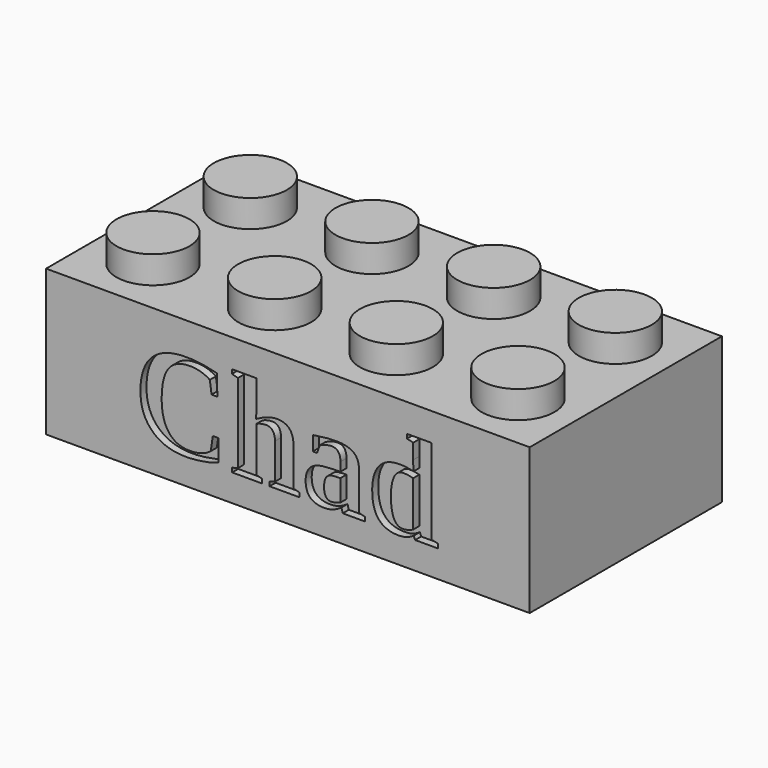
from build123d import *

# Parameters (mm, degrees)
F0_W          = 31.8
F0_H          = 15.8
F1_DEPTH      = 9.6
F2_W          = 29.4
F2_H          = 13.4
F3_DEPTH      = 8.4
F4_R          = 2.4
F5_DEPTH      = 1.8
F7_R          = 1.3
F8_DEPTH      = 1.2
F9_R          = 3.255
F9_R_2        = 2.4
F10_DEPTH     = 8.4
F11_TEXT_SIZE = 8.6100864185
F12_DEPTH     = 0.5
F13_W         = 0.6
F13_H         = 0.3
F14_DEPTH     = 8.4
F15_W         = 0.3
F15_H         = 0.6
F16_DEPTH     = 8.4
F17_W         = 0.6
F17_H         = 4
F18_DEPTH     = 6.4


# Not quite as in the source:
# - Text() gives the source's letters only with a copy of the font that has no kerning and outlines rounded to 1/6400 em; it was checked with that copy


with BuildPart() as f1:
    # F0 (on Top) → F1 (new body)
    with BuildSketch(Plane.XY):
        Rectangle(F0_W, F0_H)
    extrude(amount=F1_DEPTH)

    # F2 (on face) → F3 (cut)
    with BuildSketch(Plane.XY):
        Rectangle(F2_W, F2_H)
    extrude(amount=F3_DEPTH, mode=Mode.SUBTRACT)

    # F4 (on face) → F5 (join)
    with BuildSketch(Plane.XY.offset(9.6)):
        with Locations((-11.95, 3.95)):
            Circle(F4_R)
        with Locations((-11.95, -4.05)):
            Circle(F4_R)
        with Locations((-3.95, 3.95)):
            Circle(F4_R)
        with Locations((-3.95, -4.05)):
            Circle(F4_R)
        with Locations((4.05, 3.95)):
            Circle(F4_R)
        with Locations((4.05, -4.05)):
            Circle(F4_R)
        with Locations((12.05, 3.95)):
            Circle(F4_R)
        with Locations((12.05, -4.05)):
            Circle(F4_R)
    extrude(amount=F5_DEPTH)

    # F7 (on offset) → F8 (cut)
    with BuildSketch(Plane.XY.offset(8.4)):
        with Locations((-11.95, -3.95)):
            Circle(F7_R)
        with Locations((-11.95, 4.05)):
            Circle(F7_R)
        with Locations((-3.95, -3.95)):
            Circle(F7_R)
        with Locations((-3.95, 4.05)):
            Circle(F7_R)
        with Locations((4.05, -3.95)):
            Circle(F7_R)
        with Locations((4.05, 4.05)):
            Circle(F7_R)
        with Locations((12.05, -3.95)):
            Circle(F7_R)
        with Locations((12.05, 4.05)):
            Circle(F7_R)
    extrude(amount=F8_DEPTH, mode=Mode.SUBTRACT)

    # F9 (on offset) → F10 (join, through all)
    with BuildSketch(Plane.XY.offset(8.4)):
        with Locations((-7.95, 0.05)):
            Circle(F9_R)
        with Locations((-7.95, 0.05)):
            Circle(F9_R_2, mode=Mode.SUBTRACT)
        with Locations((0.05, 0.05)):
            Circle(F9_R)
        with Locations((0.05, 0.05)):
            Circle(F9_R_2, mode=Mode.SUBTRACT)
        with Locations((8.05, 0.05)):
            Circle(F9_R)
        with Locations((8.05, 0.05)):
            Circle(F9_R_2, mode=Mode.SUBTRACT)
    extrude(amount=-F10_DEPTH)

    # F11 (on face) → F12 (cut)
    with BuildSketch(Plane.XZ.offset(7.9)):
        with Locations((-10.1164667867, 1.779385726)):
            Text('Chad', F11_TEXT_SIZE, font='Tinos', font_style=FontStyle.BOLD, text_align=(TextAlign.LEFT, TextAlign.BOTTOM))
    extrude(amount=-F12_DEPTH, mode=Mode.SUBTRACT)

    # F13 (on face) → F14 (join, through all)
    with BuildSketch(Plane.XY):
        with Locations((-11.95, -6.55)):
            Rectangle(F13_W, F13_H)
        with Locations((-11.95, 6.55)):
            Rectangle(F13_W, F13_H)
        with Locations((-3.95, -6.55)):
            Rectangle(F13_W, F13_H)
        with Locations((-3.95, 6.55)):
            Rectangle(F13_W, F13_H)
        with Locations((4.05, -6.55)):
            Rectangle(F13_W, F13_H)
        with Locations((4.05, 6.55)):
            Rectangle(F13_W, F13_H)
        with Locations((12.05, -6.55)):
            Rectangle(F13_W, F13_H)
        with Locations((12.05, 6.55)):
            Rectangle(F13_W, F13_H)
    extrude(amount=F14_DEPTH)

    # F15 (on face) → F16 (join, through all)
    with BuildSketch(Plane.XY):
        with Locations((-14.55, -3.95)):
            Rectangle(F15_W, F15_H)
        with Locations((-14.55, 4.05)):
            Rectangle(F15_W, F15_H)
        with Locations((14.55843, -3.95)):
            Rectangle(F15_W, F15_H)
        with Locations((14.55843, 4.05)):
            Rectangle(F15_W, F15_H)
    extrude(amount=F16_DEPTH)

    # F17 (on offset) → F18 (join)
    with BuildSketch(Plane.XY.offset(8.4)):
        with Locations((0, 4.9)):
            Rectangle(F17_W, F17_H)
        with Locations((0, -4.9338)):
            Rectangle(F17_W, F17_H)
    extrude(amount=-F18_DEPTH)


solid = f1.part
